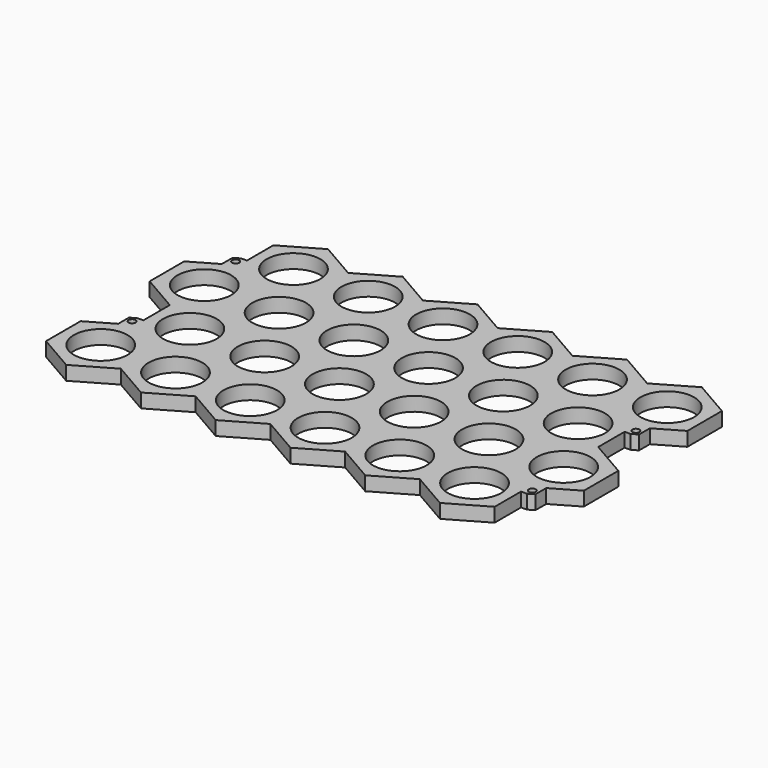
from build123d import *

# Parameters (mm, degrees)
F0_R     = 11.5
F0_R_2   = 1.5
F1_DEPTH = 6
F2_DEPTH = 6


# Not quite as in the source:
# - a feature names something its author has since deleted; it is built from what else it names


with BuildPart() as f1:
    # F0 (on Top) → F1 (new body)
    with BuildSketch(Plane.XY):
        Polygon((32, 18.4752086141), (16, 9.237604307), (16, -9.237604307), (32, -18.4752086141), (48, -9.237604307), (48, 9.237604307), align=None)
        with Locations((32, 0)):
            Circle(F0_R, mode=Mode.SUBTRACT)
        Polygon((16, -9.237604307), (16, 9.237604307), (0, 18.4752086141), (-2.5, 17.0318329411), (-5, 15.5884572681), (-16, 9.237604307), (-16, -9.237604307), (0, -18.4752086141), align=None)
        Circle(F0_R, mode=Mode.SUBTRACT)
        Polygon((0, 18.4752086141), (16, 9.237604307), (32, 18.4752086141), (32, 36.9504172281), (16, 46.1880215352), (0, 36.9504172281), (0, 22.805335633), (0, 21.36195996), align=None)
        with Locations((16, 27.7128129211)):
            Circle(F0_R, mode=Mode.SUBTRACT)
        Polygon((-2.5, 17.0318329411), (0, 18.4752086141), (0, 21.36195996), (-2.5, 22.805335633), (-5, 21.36195996), (-5, 18.4752086141), align=None)
        with Locations((-2.5, 19.918584287)):
            Circle(F0_R_2, mode=Mode.SUBTRACT)
        Polygon((32, 36.9504172281), (32, 18.4752086141), (48, 9.237604307), (64, 18.4752086141), (64, 36.9504172281), (48, 46.1880215352), align=None)
        with Locations((48, 27.7128129211)):
            Circle(F0_R, mode=Mode.SUBTRACT)
        Polygon((64, 18.4752086141), (48, 9.237604307), (48, -9.237604307), (64, -18.4752086141), (80, -9.237604307), (80, 9.237604307), align=None)
        with Locations((64, 0)):
            Circle(F0_R, mode=Mode.SUBTRACT)
        Polygon((16, 46.1880215352), (32, 36.9504172281), (48, 46.1880215352), (48, 64.6632301492), (32, 73.9008344563), (16, 64.6632301492), align=None)
        with Locations((32, 55.4256258422)):
            Circle(F0_R, mode=Mode.SUBTRACT)
        Polygon((64, 36.9504172281), (64, 18.4752086141), (80, 9.237604307), (96, 18.4752086141), (96, 36.9504172281), (80, 46.1880215352), align=None)
        with Locations((80, 27.7128129211)):
            Circle(F0_R, mode=Mode.SUBTRACT)
        Polygon((0, 36.9504172281), (16, 46.1880215352), (16, 64.6632301492), (0, 73.9008344563), (-2.5, 72.4574587833), (-5, 71.0140831103), (-16, 64.6632301492), (-16, 46.1880215352), align=None)
        with Locations((0, 55.4256258422)):
            Circle(F0_R, mode=Mode.SUBTRACT)
        Polygon((48, 64.6632301492), (48, 46.1880215352), (64, 36.9504172281), (80, 46.1880215352), (80, 64.6632301492), (64, 73.9008344563), align=None)
        with Locations((64, 55.4256258422)):
            Circle(F0_R, mode=Mode.SUBTRACT)
        Polygon((96, 18.4752086141), (80, 9.237604307), (80, -9.237604307), (96, -18.4752086141), (112, -9.237604307), (112, 9.237604307), align=None)
        with Locations((96, 0)):
            Circle(F0_R, mode=Mode.SUBTRACT)
        Polygon((32, 73.9008344563), (48, 64.6632301492), (64, 73.9008344563), (64, 92.3760430703), (48, 101.6136473774), (32, 92.3760430703), align=None)
        with Locations((48, 83.1384387633)):
            Circle(F0_R, mode=Mode.SUBTRACT)
        Polygon((96, 36.9504172281), (96, 18.4752086141), (112, 9.237604307), (128, 18.4752086141), (128, 36.9504172281), (112, 46.1880215352), align=None)
        with Locations((112, 27.7128129211)):
            Circle(F0_R, mode=Mode.SUBTRACT)
        Polygon((80, 64.6632301492), (80, 46.1880215352), (96, 36.9504172281), (112, 46.1880215352), (112, 64.6632301492), (96, 73.9008344563), align=None)
        with Locations((96, 55.4256258422)):
            Circle(F0_R, mode=Mode.SUBTRACT)
        Polygon((-2.5, 72.4574587833), (0, 73.9008344563), (0, 76.7875858022), (-2.5, 78.2309614752), (-5, 76.7875858022), (-5, 73.9008344563), align=None)
        with Locations((-2.5, 75.3442101292)):
            Circle(F0_R_2, mode=Mode.SUBTRACT)
        Polygon((64, 92.3760430703), (64, 73.9008344563), (80, 64.6632301492), (96, 73.9008344563), (96, 92.3760430703), (80, 101.6136473774), align=None)
        with Locations((80, 83.1384387633)):
            Circle(F0_R, mode=Mode.SUBTRACT)
        Polygon((128, 18.4752086141), (112, 9.237604307), (112, -9.237604307), (128, -18.4752086141), (144, -9.237604307), (144, 9.237604307), align=None)
        with Locations((128, 0)):
            Circle(F0_R, mode=Mode.SUBTRACT)
        Polygon((128, 36.9504172281), (128, 18.4752086141), (144, 9.237604307), (160, 18.4752086141), (160, 36.9504172281), (144, 46.1880215352), align=None)
        with Locations((144, 27.7128129211)):
            Circle(F0_R, mode=Mode.SUBTRACT)
        Polygon((112, 64.6632301492), (112, 46.1880215352), (128, 36.9504172281), (144, 46.1880215352), (144, 64.6632301492), (128, 73.9008344563), align=None)
        with Locations((128, 55.4256258422)):
            Circle(F0_R, mode=Mode.SUBTRACT)
        Polygon((96, 92.3760430703), (96, 73.9008344563), (112, 64.6632301492), (128, 73.9008344563), (128, 92.3760430703), (112, 101.6136473774), align=None)
        with Locations((112, 83.1384387633)):
            Circle(F0_R, mode=Mode.SUBTRACT)
        Polygon((160, 18.4752086141), (144, 9.237604307), (144, -9.237604307), (160, -18.4752086141), (176, -9.237604307), (176, 4.9074772881), (176, 6.3508529611), (176, 9.237604307), align=None)
        with Locations((160, 0)):
            Circle(F0_R, mode=Mode.SUBTRACT)
        Polygon((160, 36.9504172281), (160, 18.4752086141), (176, 9.237604307), (178.5, 10.68097998), (181, 12.124355653), (192, 18.4752086141), (192, 36.9504172281), (176, 46.1880215352), align=None)
        with Locations((176, 27.7128129211)):
            Circle(F0_R, mode=Mode.SUBTRACT)
        Polygon((144, 64.6632301492), (144, 46.1880215352), (160, 36.9504172281), (176, 46.1880215352), (176, 60.3331031303), (176, 61.7764788033), (176, 64.6632301492), (160, 73.9008344563), align=None)
        with Locations((160, 55.4256258422)):
            Circle(F0_R, mode=Mode.SUBTRACT)
        Polygon((128, 92.3760430703), (128, 73.9008344563), (144, 64.6632301492), (160, 73.9008344563), (160, 92.3760430703), (144, 101.6136473774), align=None)
        with Locations((144, 83.1384387633)):
            Circle(F0_R, mode=Mode.SUBTRACT)
        Polygon((160, 92.3760430703), (160, 73.9008344563), (176, 64.6632301492), (178.5, 66.1066058222), (181, 67.5499814952), (192, 73.9008344563), (192, 92.3760430703), (176, 101.6136473774), align=None)
        with Locations((176, 83.1384387633)):
            Circle(F0_R, mode=Mode.SUBTRACT)
    extrude(amount=F1_DEPTH)

    # F0 (on Top) → F2 (join)
    with BuildSketch(Plane.XY):
        Polygon((0, 18.4752086141), (16, 9.237604307), (32, 18.4752086141), (32, 36.9504172281), (16, 46.1880215352), (0, 36.9504172281), (0, 22.805335633), (0, 21.36195996), align=None)
        with Locations((16, 27.7128129211)):
            Circle(F0_R, mode=Mode.SUBTRACT)
        Polygon((0, 73.9008344563), (16, 64.6632301492), (32, 73.9008344563), (32, 92.3760430703), (16, 101.6136473774), (0, 92.3760430703), (0, 78.2309614752), (0, 76.7875858022), align=None)
        with Locations((16, 83.1384387633)):
            Circle(F0_R, mode=Mode.SUBTRACT)
        Polygon((178.5, 10.68097998), (176, 9.237604307), (176, 6.3508529611), (178.5, 4.9074772881), (181, 6.3508529611), (181, 9.237604307), align=None)
        with Locations((178.5, 7.7942286341)):
            Circle(F0_R_2, mode=Mode.SUBTRACT)
        Polygon((178.5, 66.1066058222), (176, 64.6632301492), (176, 61.7764788033), (178.5, 60.3331031303), (181, 61.7764788033), (181, 64.6632301492), align=None)
        with Locations((178.5, 63.2198544763)):
            Circle(F0_R_2, mode=Mode.SUBTRACT)
        Polygon((-5, 71.0140831103), (-2.5, 72.4574587833), (-5, 73.9008344563), align=None)
        Polygon((-2.5, 78.2309614752), (0, 76.7875858022), (0, 78.2309614752), align=None)
        Polygon((-2.5, 22.805335633), (0, 21.36195996), (0, 22.805335633), align=None)
        Polygon((-5, 15.5884572681), (-2.5, 17.0318329411), (-5, 18.4752086141), align=None)
        Polygon((176, 61.7764788033), (176, 60.3331031303), (178.5, 60.3331031303), align=None)
        Polygon((181, 67.5499814952), (178.5, 66.1066058222), (181, 64.6632301492), align=None)
        Polygon((178.5, 4.9074772881), (176, 6.3508529611), (176, 4.9074772881), align=None)
        Polygon((181, 12.124355653), (178.5, 10.68097998), (181, 9.237604307), align=None)
    extrude(amount=F2_DEPTH)


solid = f1.part
